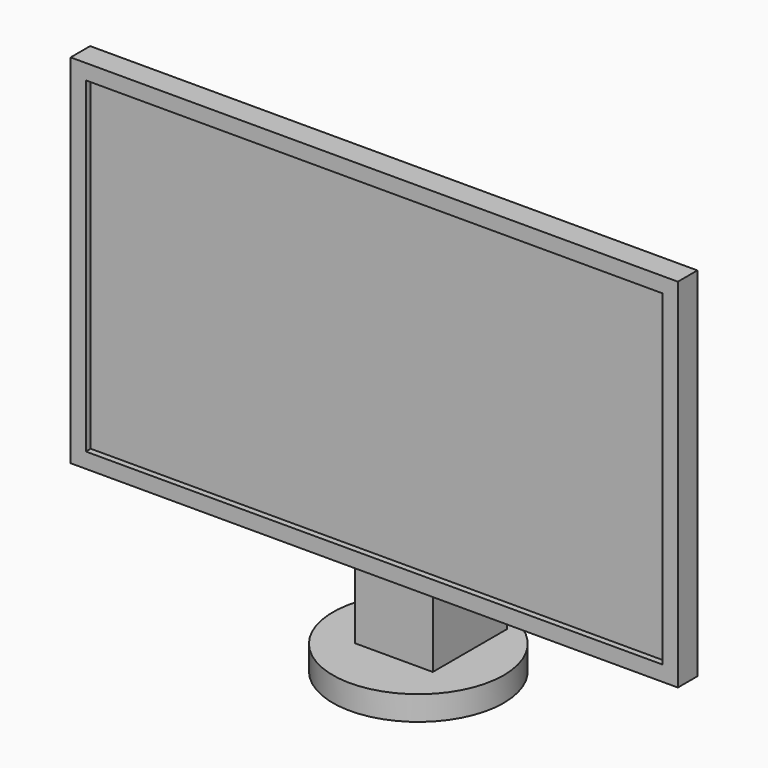
from build123d import *

# Parameters (mm, degrees)
F0_W         = 631.7488
F0_H         = 371.729
F0_W_2       = 599.9988
F0_H_2       = 339.979
F1_DEPTH     = 25.4
F2_DEPTH     = 12.7
F3_W         = 406.4
F3_H         = 209.55
F4_DEPTH     = 19.05
F5_W         = 406.4
F5_H         = 15.875
F5_H_2       = 47.625
F6_DEPTH     = 9.525
F8_DEPTH     = 9.525
F9_W         = 76.4845596125
F9_H         = 31.75
F10_DEPTH    = 44.45
F11_W        = 76.4845596125
F11_H        = 44.45
F12_DEPTH    = 101.6
F13_R        = 88.9
F14_DEPTH    = 25.4
F16_DEPTH    = 76.4845596125
F17_DEPTH    = 6.35
F18_W        = 81.1431687325
F18_H        = 148.663751781
F19_DEPTH    = 96.52
F20_T4_DEPTH = 760.4789468336
F22_DEPTH    = 81.026


# Not quite as in the source:
# - a fillet or chamfer that OpenCascade refuses, or shapes differently, is made with other operations: its cross-section is extruded or revolved along the edge and cut away or added
# - a feature names something its author has since deleted; it is built from what else it names


with BuildPart() as f1:
    # F0 (on Front) → F1 (new body)
    with BuildSketch(Plane.XZ):
        with Locations((-9.705722332, 43.6128355046)):
            Rectangle(F0_W, F0_H)
        with Locations((-9.705722332, 43.6128355046)):
            Rectangle(F0_W_2, F0_H_2, mode=Mode.SUBTRACT)
    extrude(amount=F1_DEPTH)

    # F0 (on Front) → F2 (join)
    with BuildSketch(Plane.XZ):
        with Locations((-9.705722332, 43.6128355046)):
            Rectangle(F0_W_2, F0_H_2)
    extrude(amount=F2_DEPTH)

    # F3 (on face) → F4 (join)
    with BuildSketch(Plane.XZ):
        with Locations((-9.705722332, 26.0233355046)):
            Rectangle(F3_W, F3_H)
    extrude(amount=-F4_DEPTH)

    # F5 (on face) → F6 (cut)
    with BuildSketch(Plane.XZ):
        with Locations((-9.705722332, -134.3141644954)):
            Rectangle(F5_W, F5_H)
        with Locations((-9.705722332, -102.5641644954)):
            Rectangle(F5_W, F5_H_2)
    extrude(amount=F6_DEPTH, mode=Mode.SUBTRACT)

    # F7 (on face) → F8 (join)
    with BuildSketch(Plane.XZ):
        Polygon((-50.980722332, -126.3766644954), (31.569277668, -126.3766644954), (31.9963085321, -78.7516644954), (31.569277668, -78.7516644954), (-50.980722332, -78.7516644954), align=None)
    extrude(amount=-F8_DEPTH)

    # F9 (on face) → F10 (join)
    with BuildSketch(Plane(origin=(0, 9.525, 0), x_dir=(-1, 0, 0), z_dir=(0, 1, 0))):
        with Locations((9.5634425258, -110.5016644954)):
            Rectangle(F9_W, F9_H)
    extrude(amount=F10_DEPTH)

    # F11 (on face) → F12 (join)
    with BuildSketch(Plane(origin=(0, 0, -126.3766644954), x_dir=(1, 0, 0), z_dir=(0, 0, -1))):
        with Locations((-9.5634425258, -31.75)):
            Rectangle(F11_W, F11_H)
    extrude(amount=F12_DEPTH)

    # F15 (on face) → F16 (cut, through all)
    with BuildSketch(Plane(origin=(-47.805722332, 0, 0), x_dir=(0, -1, 0), z_dir=(-1, 0, 0))):
        Polygon((-9.525, -126.3766644954), (-9.525, -94.6266644954), (-53.975, -94.6266644954), (-53.975, -227.9766644954), (-9.525, -227.9766644954), align=None)
    extrude(amount=-F16_DEPTH, mode=Mode.SUBTRACT)


with BuildPart() as f14:
    # F13 (on face) → F14 (new body)
    with BuildSketch(Plane(origin=(0, 0, -227.9766644954), x_dir=(1, 0, 0), z_dir=(0, 0, -1))):
        with Locations((-9.5634425258, -31.75)):
            Circle(F13_R)
    extrude(amount=F14_DEPTH)


with BuildPart() as f17:
    # F17 (new): a face of the model
    f17_faces = [f1.part.faces().sort_by_distance(p)[0] for p in [
        (-9.705722332, -12.7, 43.6128355046),
    ]]
    extrude(f17_faces, amount=F17_DEPTH)


with BuildPart() as f1_1:
    add(f1.part)

    # F18 (on Front) → F19 (join)
    with BuildSketch(Plane.XZ):
        with Locations((-9.7057269886, -153.5059846938)):
            Rectangle(F18_W, F18_H)
    extrude(amount=-F19_DEPTH)

    # F20: chamfer of 132.08 on 1 edges, made by hand


with BuildPart() as f20_tool2:
    # F20_s3 → F20_t4 (new body)
    with BuildSketch(Plane.YZ.offset(370.5337464282)):
        Polygon((-35.56, -79.1741088033), (96.52, -211.2541088033), (96.52, -79.1741088033), align=None)
    extrude(amount=-F20_T4_DEPTH)

    split(bisect_by=Plane.XZ.offset(-9.525), keep=Keep.BOTTOM)


with BuildPart() as f1_2:
    add(f1_1.part)

    # F20_t1: cut F20_tool2
    add(f20_tool2.part, mode=Mode.SUBTRACT)

    # F21 (on face) → F22 (join)
    with BuildSketch(Plane.YZ.offset(30.8658573776)):
        Polygon((41.4450243115, -78.2184153795), (0, -78.2184153795), (0, -126.3766644954), (9.525, -126.3766644954), (9.525, -124.2591088033), (41.4450243115, -156.1791331148), align=None)
    extrude(amount=-F22_DEPTH)


solid = Compound([f14.part, f17.part, f1_2.part])
